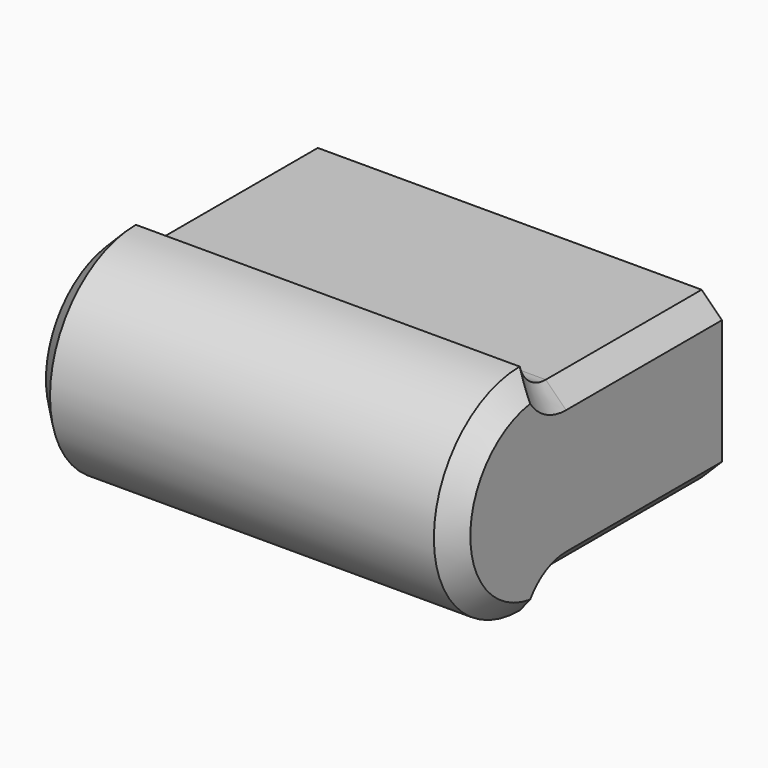
from build123d import *

# Parameters (mm, degrees)
F4_DEPTH      = 0.8
F4_DEPTH_BACK = 36.9
F5_DEPTH      = 36.1
F6_T1_DEPTH   = 37.7
F7_SIZE       = 1.8
F8_SIZE       = 1.8


# Not quite as in the source:
# - a fillet or chamfer that OpenCascade refuses, or shapes differently, is made with other operations: its cross-section is extruded or revolved along the edge and cut away or added


with BuildPart() as f4:
    # F3 (on Right) → F4 (new body, two sides)
    with BuildSketch(Plane.YZ) as f4_sk:
        with BuildLine():
            Line((20.2, 6.5358882766), (0, 6.5358882766))
            ThreePointArc((0, 6.5358882766), (-6.5358882766, 0), (0, -6.5358882766))
            Line((0, -6.5358882766), (20.2, -6.5358882766))
            Line((20.2, -6.5358882766), (20.2, 6.5358882766))
        make_face()
        with BuildLine():
            ThreePointArc((0, -6.5358882766), (-6.5358882766, 0), (0, 6.5358882766))
            Line((0, 6.5358882766), (20.2, 6.5358882766))
            Line((20.2, 6.5358882766), (20.2, 7.3358882766))
            Line((20.2, 7.3358882766), (0, 7.3358882766))
            Line((0, 7.3358882766), (0, 9.5358882766))
            ThreePointArc((0, 9.5358882766), (-9.5358882766, 0), (0, -9.5358882766))
            Line((0, -9.5358882766), (0, -7.3358882766))
            Line((0, -7.3358882766), (20.2, -7.3358882766))
            Line((20.2, -7.3358882766), (20.2, -6.5358882766))
            Line((20.2, -6.5358882766), (0, -6.5358882766))
        make_face()
    extrude(amount=-F4_DEPTH)
    extrude(f4_sk.sketch, amount=F4_DEPTH_BACK)

    # F3 (on Right) → F5 (cut)
    with BuildSketch(Plane.YZ):
        with BuildLine():
            Line((20.2, 6.5358882766), (0, 6.5358882766))
            ThreePointArc((0, 6.5358882766), (-6.5358882766, 0), (0, -6.5358882766))
            Line((0, -6.5358882766), (20.2, -6.5358882766))
            Line((20.2, -6.5358882766), (20.2, 6.5358882766))
        make_face()
    extrude(amount=F5_DEPTH, mode=Mode.SUBTRACT)

    # F6: fillet of radius 3 on 2 edges, made by hand

    # F6_s2 → F6_t1 (join)
    with BuildSketch(Plane.YZ.offset(-0.8)):
        with BuildLine():
            ThreePointArc((2.891366459, 7.3358882766), (1.0747762465, 7.9484209993), (0, 9.5358882766))
            Line((0, 9.5358882766), (0, 7.3358882766))
            Line((0, 7.3358882766), (2.891366459, 7.3358882766))
        make_face()
        with BuildLine():
            ThreePointArc((0, -9.5358882766), (1.0747762465, -7.9484209993), (2.891366459, -7.3358882766))
            Line((2.891366459, -7.3358882766), (0, -7.3358882766))
            Line((0, -7.3358882766), (0, -9.5358882766))
        make_face()
    extrude(amount=F6_T1_DEPTH)

    # F7
    f7_edges = [f4.edges().sort_by_distance(p)[0] for p in [
        (36.1, 10.1, 6.535888),
        (0, -6.535888, 0),
    ]]
    chamfer(f7_edges, length=F7_SIZE)

    # F8
    f8_edges = [f4.edges().sort_by_distance(p)[0] for p in [
        (36.9, 11.545683, 7.335888),
        (36.9, 1.074776, 7.948421),
        (36.9, -9.535888, 0),
        (36.9, 1.074776, -7.948421),
        (36.9, 11.545683, -7.335888),
        (-0.8, 11.545683, 7.335888),
        (-0.8, 1.074776, 7.948421),
        (-0.8, -9.535888, 0),
        (-0.8, 1.074776, -7.948421),
        (-0.8, 11.545683, -7.335888),
    ]]
    chamfer(f8_edges, length=F8_SIZE)


solid = f4.part
